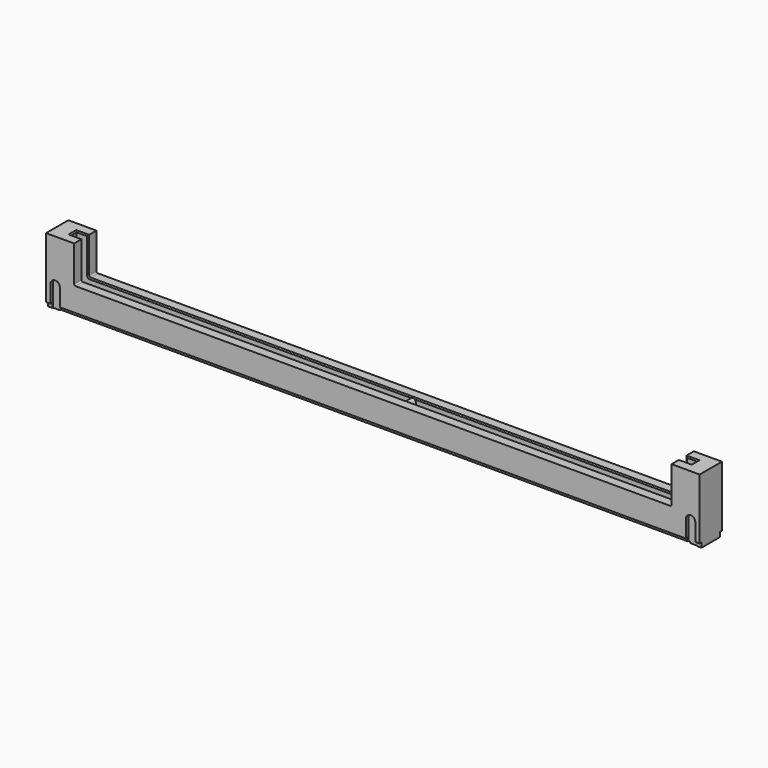
from build123d import *

# Parameters (mm, degrees)
F13_DEPTH     = 3
F0_DEPTH      = 0.65
F2_W          = 2.725
F2_H          = 0.25
F3_DEPTH      = 1.3
F4_W          = 0.5
F4_H          = 1
F5_DEPTH      = 70.401
F5_DEPTH_BACK = 70.401
F6_W          = 133.75
F6_H          = 1.58
F7_DEPTH      = 11.8
F8_R          = 0.3
F9_SIZE       = 0.25
F11_DEPTH     = 1


# Not quite as in the source:
# - a pattern or mirror of a feature is missing from the dataset's text; its kind, count and spacing are read off the source's solid


with BuildPart() as f13:
    # F12 (on Front) → F13 (new body, symmetric)
    with BuildSketch(Plane.XZ):
        Polygon((-67.9, 0), (-67.9, 0.25), (1.575, 0.25), (1.575, 0), (4.3, 0), (4.3, 0.25), (67.9, 0.25), (67.9, 0), (70.4, 0), (70.4, 14.1), (64.35, 14.1), (64.35, 6.1), (-64.35, 6.1), (-64.35, 14.1), (-70.4, 14.1), (-70.4, 0), align=None)
    extrude(amount=F13_DEPTH, both=True)

    # F15: F0, F0b across plane


with BuildPart() as f0:
    # F14 (on face) → F0 (new body)
    with BuildSketch(Plane.XZ.offset(3)):
        with BuildLine():
            Line((-69.465, 4.75), (-69.465, 0))
            Line((-69.465, 0), (-67.9, 0))
            Line((-67.9, 0), (-67.9, 0.25))
            Line((-67.9, 0.25), (-67.435, 0.25))
            Line((-67.435, 0.25), (-67.435, 4.75))
            ThreePointArc((-67.435, 4.75), (-68.45, 5.765), (-69.465, 4.75))
        make_face()
    extrude(amount=-F0_DEPTH)


with BuildPart() as f0b:
    # F14 (on face) → F0, piece 2 (new body)
    with BuildSketch(Plane.XZ.offset(3)):
        with BuildLine():
            Line((67.9, 0.25), (67.9, 0))
            Line((67.9, 0), (69.465, 0))
            Line((69.465, 0), (69.465, 4.75))
            ThreePointArc((69.465, 4.75), (68.45, 5.765), (67.435, 4.75))
            Line((67.435, 4.75), (67.435, 0.25))
            Line((67.435, 0.25), (67.9, 0.25))
        make_face()
    extrude(amount=-F0_DEPTH)


with BuildPart() as f13_1:
    add(f13.part)
    add(f0.part.mirror(Plane.XZ), mode=Mode.SUBTRACT)
    add(f0b.part.mirror(Plane.XZ), mode=Mode.SUBTRACT)

    # F1: cut F0, F0b
    add(f0.part, mode=Mode.SUBTRACT)
    add(f0b.part, mode=Mode.SUBTRACT)

    # F2 (on face) → F3 (cut)
    with BuildSketch(Plane.XZ.offset(3)):
        with Locations((2.9375, 0.125)):
            Rectangle(F2_W, F2_H)
    f3 = extrude(amount=-F3_DEPTH, mode=Mode.SUBTRACT)

    # F3_copies: F3 across plane
    add(f3.mirror(Plane.ZX), mode=Mode.SUBTRACT)

    # F4 (on Right) → F5 (cut, two sides)
    with BuildSketch(Plane.YZ) as f5_sk:
        with Locations((-2.75, 0.5)):
            Rectangle(F4_W, F4_H)
        with Locations((2.75, 0.5)):
            Rectangle(F4_W, F4_H)
    extrude(amount=-F5_DEPTH, mode=Mode.SUBTRACT)
    extrude(f5_sk.sketch, amount=F5_DEPTH_BACK, mode=Mode.SUBTRACT)

    # F6 (on face) → F7 (cut)
    with BuildSketch(Plane.XY.offset(14.1)):
        Rectangle(F6_W, F6_H)
    extrude(amount=-F7_DEPTH, mode=Mode.SUBTRACT)

    # F8
    f8_edges = [f13_1.edges().sort_by_distance(p)[0] for p in [
        (-64.35, 1.895, 6.1),
        (-64.35, -1.895, 6.1),
        (64.35, 1.895, 6.1),
        (64.35, -1.895, 6.1),
    ]]
    fillet(f8_edges, radius=F8_R)

    # F9
    f9_edges = [f13_1.edges().sort_by_distance(p)[0] for p in [
        (-65.6125, 0.79, 14.1),
        (-66.875, 0, 14.1),
        (-65.6125, -0.79, 14.1),
        (-64.35, 0.79, 10.25),
        (-64.35, -0.79, 10.25),
        (65.6125, 0.79, 14.1),
        (66.875, 0, 14.1),
        (65.6125, -0.79, 14.1),
        (-64.262132, -0.79, 6.187868),
        (0, -0.79, 6.1),
        (64.262132, -0.79, 6.187868),
        (64.35, -0.79, 10.25),
        (64.35, 0.79, 10.25),
        (64.262132, 0.79, 6.187868),
        (0, 0.79, 6.1),
        (-64.262132, 0.79, 6.187868),
    ]]
    chamfer(f9_edges, length=F9_SIZE)

    # F10 (on Front) → F11 (join, symmetric)
    with BuildSketch(Plane.XZ):
        with BuildLine():
            Line((6.275, 2.3), (6.275, 5.247))
            ThreePointArc((6.275, 5.247), (5.575, 5.947), (4.875, 5.247))
            Line((4.875, 5.247), (4.875, 2.3))
            Line((4.875, 2.3), (6.275, 2.3))
        make_face()
    extrude(amount=F11_DEPTH, both=True)


solid = f13_1.part
